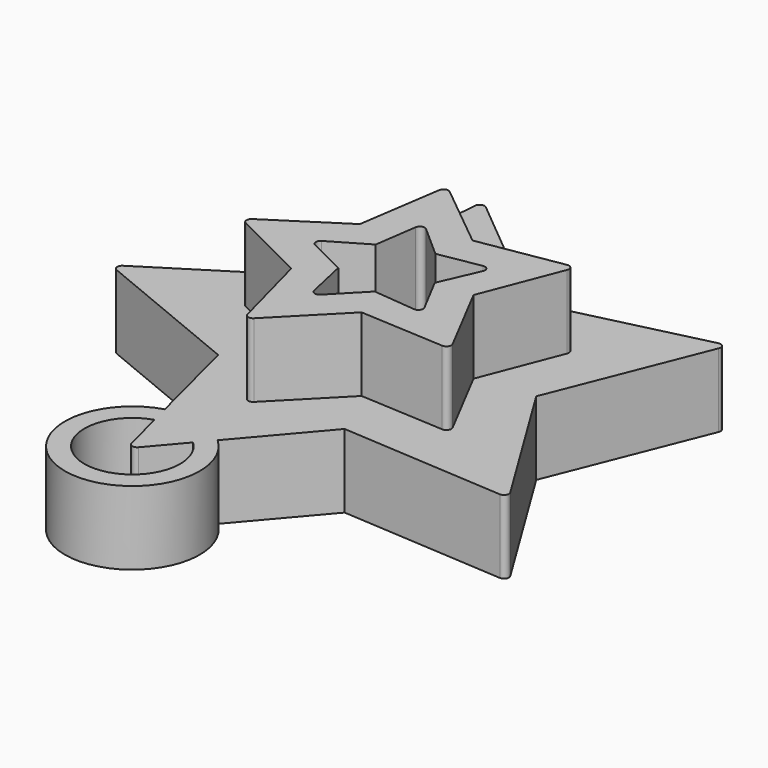
from build123d import *

# Parameters (mm, degrees)
F1_DEPTH  = 7.62
F3_DEPTH  = 7.62
F5_DEPTH  = 7.62
F8_DEPTH  = 7.62
F10_DEPTH = 7.62
F12_DEPTH = 7.62


# Not quite as in the source:
# - a feature names something its author has since deleted; it is built from what else it names


with BuildPart() as f1:
    # F0 (on Top) → F1 (new body)
    with BuildSketch(Plane.XY):
        with BuildLine():
            Line((5.2457718421, 22.65034753), (-16.6286527122, 42.176813326))
            ThreePointArc((-16.6286527122, 42.176813326), (-17.1554325452, 42.2695789476), (-17.4732486395, 41.8393518177))
            Line((-17.4732486395, 41.8393518177), (-19.9207279669, 11.9883678087))
            Line((-19.9207279669, 11.9883678087), (-45.2510694319, -2.7814364328))
            ThreePointArc((-45.2510694319, -2.7814364328), (-45.5020787015, -3.2537676721), (-45.1911189603, -3.6889762341))
            Line((-45.1911189603, -3.6889762341), (-17.5574588063, -15.2411287545))
            Line((-17.5574588063, -15.2411287545), (-11.338046224, -43.895835579))
            ThreePointArc((-11.338046224, -43.895835579), (-10.9663986511, -44.2805179605), (-10.4563988677, -44.1192645141))
            Line((-10.4563988677, -44.1192645141), (9.0696216685, -21.4079034059))
            Line((9.0696216685, -21.4079034059), (38.2437714994, -24.3476819196))
            ThreePointArc((38.2437714994, -24.3476819196), (38.724471601, -24.1130974669), (38.7287090602, -23.5782287943))
            Line((38.7287090602, -23.5782287943), (23.1627932625, 2.0103168218))
            Line((23.1627932625, 2.0103168218), (34.9739968686, 28.8481406054))
            ThreePointArc((34.9739968686, 28.8481406054), (34.8994382969, 29.3778041519), (34.3920574073, 29.5471177247))
            Line((34.3920574073, 29.5471177247), (5.2457718421, 22.65034753))
        make_face()
    extrude(amount=F1_DEPTH)

    # F2 (on face) → F3 (join)
    with BuildSketch(Plane.XY.offset(7.62)):
        with BuildLine():
            Line((-10.7096949682, 24.1632334685), (-12.0244422161, 7.2461689852))
            Line((-12.0244422161, 7.2461689852), (-26.367554987, -1.8197422817))
            ThreePointArc((-26.367554987, -1.8197422817), (-26.6022582168, -2.2927760227), (-26.2900783947, -2.7186754062))
            Line((-26.2900783947, -2.7186754062), (-10.6072732242, -9.1967347639))
            Line((-10.6072732242, -9.1967347639), (-6.4173448361, -25.6393662796))
            ThreePointArc((-6.4173448361, -25.6393662796), (-6.0399903009, -26.0087577805), (-5.5384670466, -25.8434672739))
            Line((-5.5384670466, -25.8434672739), (5.4687868356, -12.9300636548))
            Line((5.4687868356, -12.9300636548), (22.4014177608, -14.026257529))
            ThreePointArc((22.4014177608, -14.026257529), (22.8693389191, -13.7815202908), (22.8671175143, -13.2534657562))
            Line((22.8671175143, -13.2534657562), (13.9871693659, 1.2055159485))
            Line((13.9871693659, 1.2055159485), (20.2621824084, 16.9706623917))
            ThreePointArc((20.2621824084, 16.9706623917), (20.1740190532, 17.4913098242), (19.6711228952, 17.6523749678))
            Line((19.6711228952, 17.6523749678), (3.1757592389, 13.675113485))
            Line((3.1757592389, 13.675113485), (-9.8787003461, 24.5147036987))
            ThreePointArc((-9.8787003461, 24.5147036987), (-10.4011094545, 24.5917442699), (-10.7096949682, 24.1632334685))
        make_face()
    extrude(amount=F3_DEPTH)

    # F4 (on face) → F5 (join)
    with BuildSketch(Plane.XY.offset(15.24)):
        with BuildLine():
            ThreePointArc((-4.7045563215, 13.3742015157), (-5.2088793669, 13.454135563), (-5.5278964741, 13.0554385961))
            Line((-5.5278964741, 13.0554385961), (-6.8203753298, 4.4014452639))
            Line((-6.8203753298, 4.4014452639), (-14.1734093561, -0.3414433913))
            ThreePointArc((-14.1734093561, -0.3414433913), (-14.4052755444, -0.7963821309), (-14.1246739036, -1.2229895678))
            Line((-14.1246739036, -1.2229895678), (-6.2936350842, -5.1264410146))
            Line((-6.2936350842, -5.1264410146), (-4.0550923971, -13.5852251368))
            ThreePointArc((-4.0550923971, -13.5852251368), (-3.6940705368, -13.946326788), (-3.2016320784, -13.811287717))
            Line((-3.2016320784, -13.811287717), (2.9306949349, -7.5697600522))
            Line((2.9306949349, -7.5697600522), (11.6672244272, -8.0546874881))
            ThreePointArc((11.6672244272, -8.0546874881), (12.1222143958, -7.8229218423), (12.1459564597, -7.3128556696))
            Line((12.1459564597, -7.3128556696), (8.1049041646, 0.4480720157))
            Line((8.1049041646, 0.4480720157), (11.2658336475, 8.6071545004))
            ThreePointArc((11.2658336475, 8.6071545004), (11.1860110523, 9.1114951981), (10.7082459963, 9.2916943583))
            Line((10.7082459963, 9.2916943583), (2.0784113144, 7.8466837873))
            Line((2.0784113144, 7.8466837873), (-4.7045563215, 13.3742015157))
        make_face()
    extrude(amount=F5_DEPTH)

    # F8 (cut): a face of the model
    f8_faces = [f1.faces().sort_by_distance(p)[0] for p in [
        (0, 0, 0),
    ]]
    extrude(f8_faces, amount=-F8_DEPTH, mode=Mode.SUBTRACT)

    # F9 (on face) → F10 (cut)
    with BuildSketch(Plane.XY.offset(22.86)):
        with BuildLine():
            ThreePointArc((-2.1197789922, 7.0861071574), (-2.6315872512, 7.1830271414), (-2.9596514058, 6.77840993))
            Line((-2.9596514058, 6.77840993), (-3.5885418896, 2.4094997361))
            Line((-3.5885418896, 2.4094997361), (-7.3943361202, 0.173697912))
            ThreePointArc((-7.3943361202, 0.173697912), (-7.6446699524, -0.2831107457), (-7.3612335158, -0.7201518922))
            Line((-7.3612335158, -0.7201518922), (-3.400490854, -2.6683297817))
            Line((-3.400490854, -2.6683297817), (-2.4501720543, -6.9787559441))
            ThreePointArc((-2.4501720543, -6.9787559441), (-2.0930786121, -7.3579992049), (-1.5898411061, -7.2234882764))
            Line((-1.5898411061, -7.2234882764), (1.4869229634, -4.0586182344))
            Line((1.4869229634, -4.0586182344), (5.8800465123, -4.4868062846))
            ThreePointArc((5.8800465123, -4.4868062846), (6.351076229, -4.2643828521), (6.3786576755, -3.7442093799))
            Line((6.3786576755, -3.7442093799), (4.319459784, 0.1599657655))
            Line((4.319459784, 0.1599657655), (6.0842406543, 4.2057571592))
            ThreePointArc((6.0842406543, 4.2057571592), (6.0182595868, 4.7224656612), (5.5320683522, 4.9094396186))
            Line((5.5320683522, 4.9094396186), (1.1826499962, 4.1574825145))
            Line((1.1826499962, 4.1574825145), (-2.1197789922, 7.0861071574))
        make_face()
    extrude(amount=-F10_DEPTH, mode=Mode.SUBTRACT)

    # F11 (on face) → F12 (join)
    with BuildSketch(Plane(origin=(0, 0, 7.62), x_dir=(1, 0, 0), z_dir=(0, 0, -1))):
        with BuildLine():
            Line((-2.6220134118, 22.4219651148), (-1.3098667841, 20.8825912445))
            ThreePointArc((-1.3098667841, 20.8825912445), (-7.6178176155, 32.8030283673), (-8.0269681328, 19.3226848722))
            Line((-8.0269681328, 19.3226848722), (-7.5274974689, 21.282768988))
            ThreePointArc((-7.5274974689, 21.282768988), (-7.1607580244, 30.8348874257), (-2.6220134118, 22.4219651148))
        make_face()
    extrude(amount=-F12_DEPTH)


solid = f1.part
